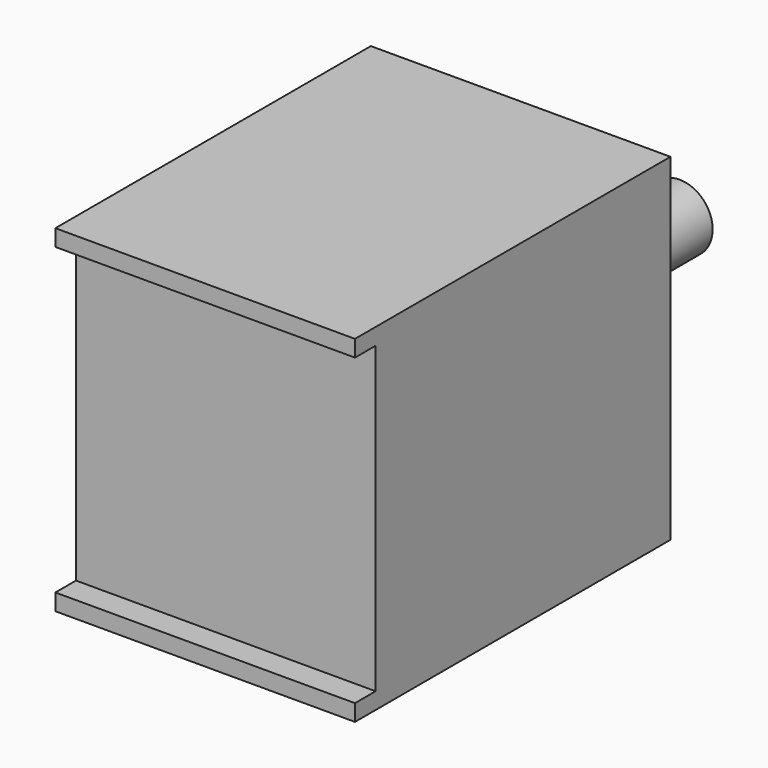
from build123d import *

# Parameters (mm, degrees)
F1_DEPTH = 67.4566328526
F2_DEPTH = 6.2197912484
F4_DEPTH = 12.4627631158


with BuildPart() as f1:
    # F0 (on Right) → F1 (new body)
    with BuildSketch(Plane.YZ):
        Polygon((-5.8088302612, 34.2432931066), (0, 34.2432931066), (0, -34.2432931066), (-5.8088302612, -34.2432931066), (-5.8088302612, -37.9646643996), (76.7590999603, -37.9646643996), (76.7590999603, 37.9646643996), (-5.8088302612, 37.9646643996), align=None)
    extrude(amount=F1_DEPTH)

    # F2 (add): a face of the model
    f2_faces = [f1.faces().sort_by_distance(p)[0] for p in [
        (33.7283164263, 76.7590999603, 0),
    ]]
    extrude(f2_faces, amount=F2_DEPTH)

    # F3 (on face) → F4 (join)
    with BuildSketch(Plane(origin=(0, 82.9788912088, 0), x_dir=(-1, 0, 0), z_dir=(0, 1, 0))):
        with BuildLine():
            ThreePointArc((-38.3854716222, 0.9479600765), (-36.6591605512, 5.8587284108), (-37.6652367413, 10.9659396112))
            ThreePointArc((-37.6652367413, 10.9659396112), (-40.901393767, 22.4123427927), (-52.0788472287, 18.3432652315))
            ThreePointArc((-52.0788472287, 18.3432652315), (-65.9917417473, 22.0669934876), (-55.7989236075, 11.8914716641))
            Line((-55.7989236075, 11.8914716641), (-55.7989236075, 0))
            Line((-55.7989236075, 0), (-50.582356751, 6.5680034459))
            Line((-50.582356751, 6.5680034459), (-46.5246960521, 6.5680034459))
            ThreePointArc((-46.5246960521, 6.5680034459), (-44.599657899, 1.9303920858), (-44.8609884943, -3.0840787076))
            Line((-44.8609884943, -3.0840787076), (-38.3854716222, 0.9479600765))
        make_face()
    extrude(amount=F4_DEPTH)


solid = f1.part
